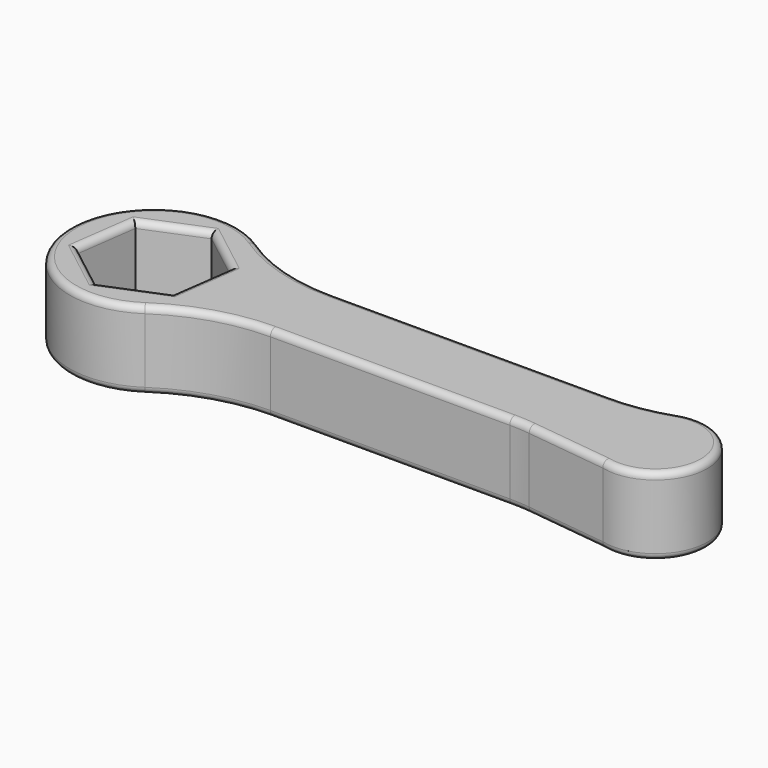
from build123d import *

# Parameters (mm, degrees)
F1_DEPTH    = 6
F2_R        = 14
F3_T1_DEPTH = 6
F4_R        = 13
F5_R        = 0.5


# Not quite as in the source:
# - a fillet or chamfer that OpenCascade refuses, or shapes differently, is made with other operations: its cross-section is extruded or revolved along the edge and cut away or added


with BuildPart() as f1:
    # F0 (on Top) → F1 (new body)
    with BuildSketch(Plane.XY):
        with BuildLine():
            Line((36.1013870801, 3.026675175), (5.7523245202, 3.026675175))
            ThreePointArc((5.7523245202, 3.026675175), (-6.5, 0), (5.7523245202, -3.026675175))
            Line((5.7523245202, -3.026675175), (36.1013870801, -3.026675175))
            ThreePointArc((36.1013870801, -3.026675175), (42.7283578295, 0), (36.1013870801, 3.026675175))
        make_face()
        Polygon((-3.7867383436, 2.9366555893), (0.6498491707, 4.7477393977), (4.4365875143, 1.8110838084), (3.7867383436, -2.9366555893), (-0.6498491707, -4.7477393977), (-4.4365875143, -1.8110838084), align=None, mode=Mode.SUBTRACT)
    extrude(amount=F1_DEPTH)

    # F2
    f2_edges = [f1.edges().sort_by_distance(p)[0] for p in [
        (5.752325, -3.026675, 3),
        (5.752325, 3.026675, 3),
        (36.101387, 3.026675, 3),
    ]]
    fillet(f2_edges, radius=F2_R)

    # F3: chamfer of 11 on 1 edges, made by hand

    # F3_s2 → F3_t1 (join)
    with BuildSketch(Plane.XY):
        with BuildLine():
            Line((30.2515384912, -2.9735152662), (38.1998957411, -3.9409061384))
            Line((38.1998957411, -3.9409061384), (38.2526662364, -3.7273288109))
            ThreePointArc((38.2526662364, -3.7273288109), (37.1662038799, -3.4493250658), (36.2454465167, -2.8604016692))
            Line((36.2454465167, -2.8604016692), (36.1013870801, -2.806675175))
            ThreePointArc((36.1013870801, -2.806675175), (33.1764627857, -2.806675175), (30.2515384912, -2.7535152662))
            Line((30.2515384912, -2.7535152662), (30.2515384912, -2.9735152662))
        make_face()
    extrude(amount=F3_T1_DEPTH)

    # F4
    f4_edges = [f1.edges().sort_by_distance(p)[0] for p in [
        (30.688315, -3.026675, 3),
    ]]
    fillet(f4_edges, radius=F4_R)

    # F5
    f5_edges = [f1.edges().sort_by_distance(p)[0] for p in [
        (20.658434, -3.026675, 0),
        (30.686871, -3.050504, 0),
        (7.341933, -3.632803, 0),
        (34.616932, -3.504825, 0),
        (-6.5, 0, 0),
        (42.724404, 0.177915, 0),
        (7.341933, 3.632803, 0),
        (35.177697, 3.218098, 0),
        (22.143624, 3.026675, 0),
        (-4.111663, 0.562786, 0),
        (-1.568445, 3.842197, 0),
        (2.543218, 3.279412, 0),
        (4.111663, -0.562786, 0),
        (1.568445, -3.842197, 0),
        (-2.543218, -3.279412, 0),
        (20.658434, -3.026675, 6),
        (30.686871, -3.050504, 6),
        (7.341933, -3.632803, 6),
        (34.616932, -3.504825, 6),
        (-6.5, 0, 6),
        (42.724404, 0.177915, 6),
        (7.341933, 3.632803, 6),
        (35.177697, 3.218098, 6),
        (22.143624, 3.026675, 6),
        (-4.111663, 0.562786, 6),
        (-1.568445, 3.842197, 6),
        (2.543218, 3.279412, 6),
        (4.111663, -0.562786, 6),
        (1.568445, -3.842197, 6),
        (-2.543218, -3.279412, 6),
    ]]
    fillet(f5_edges, radius=F5_R)


solid = f1.part
